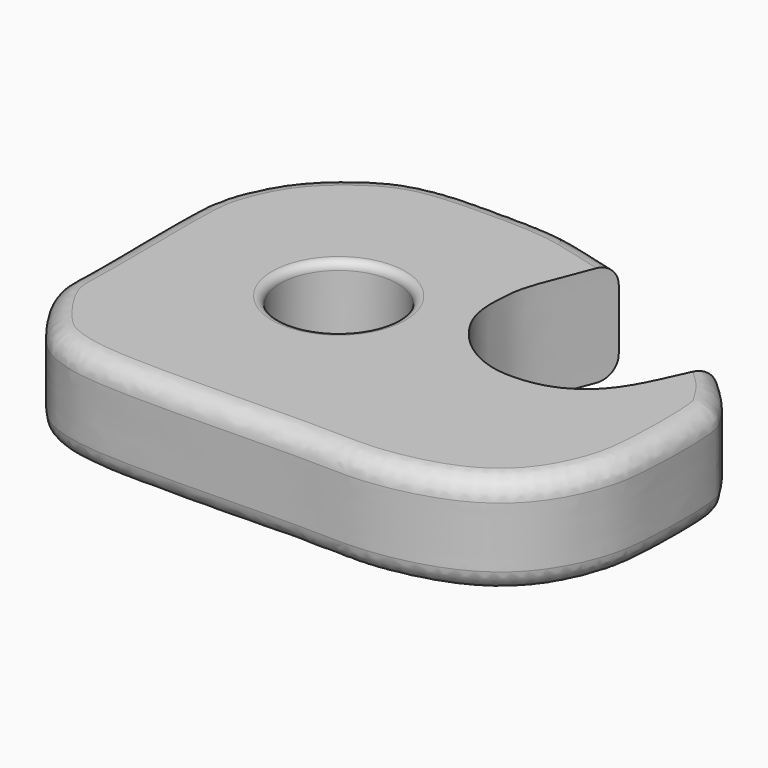
from build123d import *

# Parameters (mm, degrees)
F0_R     = 14.4754712181
F1_DEPTH = 25
F2_R     = 5
F3_R     = 2


with BuildPart() as f1:
    # F0 (on Top) → F1 (new body)
    with BuildSketch(Plane.XY):
        with BuildLine():
            add(Edge.make_bspline(
                [(4.7748561241, 37.0201033496), (1.8727595404, 29.1179646637), (-2.9520116751, 17.9431651207), (-3.3954410177, 12.5793787294), (-3.8071188973, 7.0032014822), (-2.9373384689, 1.6316462754), (-0.6202760255, -2.674310752), (2.3822429436, -6.5357445519), (6.1668697528, -9.7114229849), (10.602603783, -12.05921425), (15.8641316415, -13.4566744805), (22.5388029859, -13.2153438488), (28.2399223964, -11.6976770266), (33.1166668127, -8.7165652858), (36.6710528234, -5.1063898982), (40.3178554583, 0.2360357339), (44.1224099682, 9.0600683626), (46.6542359817, 14.6099540463)],
                knots=[0, 0, 0, 0, 0.1184466174, 0.1765135306, 0.2361345285, 0.2963530059, 0.3530939828, 0.4100083101, 0.4672157798, 0.5246310732, 0.5847048161, 0.651176237, 0.7141127993, 0.775218742, 0.8320476108, 0.8962180189, 1, 1, 1, 1], degree=3))
            add(Edge.make_bspline(
                [(47.3992715806, 14.408958469), (49.5581893602, 12.4293635752), (53.0552771378, 9.14091091), (55.873000337, 4.1728539766), (58.0743199218, 1.4042803534), (57.860107885, -21.4624474724), (56.0155753338, -30.8248650048), (50.6028118678, -43.2032629444), (38.5946445224, -53.9006460259), (17.5542269329, -58.7848208722), (1.8947153131, -57.2572408539), (-48.4788210559, -59.4518328809), (-60.1063658028, -55.7026316627), (-65.7202395809, -52.887305593), (-75.7818557148, -39.1486573699), (-74.5109896884, -29.1899746736), (-75.5520721833, 5.2121806053), (-73.7558927727, 13.4740548272), (-68.2744464695, 26.2721216828), (-56.4052432789, 36.1092530167), (-48.4018948612, 39.8969175531), (-40.2520257831, 41.5180153708), (-29.7568874334, 41.8111730776), (-19.7296486967, 41.7643519531), (-9.3130325779, 41.1205361444), (-0.2326000752, 38.2673542099), (4.7748561241, 37.0201033496)],
                knots=[0, 0, 0, 0, 0.0326111141, 0.0587556715, 0.0801046744, 0.133814265, 0.1716835185, 0.2121781721, 0.2581911555, 0.3094700605, 0.3580706974, 0.4393602896, 0.4787102265, 0.5065811362, 0.5514958373, 0.5903021331, 0.6566719682, 0.6916657518, 0.7331790655, 0.7783952394, 0.8123276102, 0.8450064218, 0.8823187216, 0.9187526227, 0.9556883694, 1, 1, 1, 1], degree=3))
            add(Edge.make_bspline(
                [(46.6542359817, 14.6099540463), (46.7139919849, 14.7342493796), (47.3395155774, 14.2846631356), (47.3992715806, 14.408958469)],
                knots=[0, 0, 0, 0, 0.7716717345, 0.7716717345, 0.7716717345, 0.7716717345], degree=3))
        make_face()
        with Locations((-28.6872740835, -7.8522199765)):
            Circle(F0_R, mode=Mode.SUBTRACT)
    extrude(amount=F1_DEPTH)

    # F2
    f2_edges = [f1.edges().sort_by_distance(p)[0] for p in [
        (-55.074943, -57.039955, 25),
        (-55.074943, -57.039955, 0),
    ]]
    fillet(f2_edges, radius=F2_R)

    # F3
    f3_edges = [f1.edges().sort_by_distance(p)[0] for p in [
        (-14.211803, -7.85222, 12.5),
        (-43.162745, -7.85222, 0),
        (-43.162745, -7.85222, 25),
    ]]
    fillet(f3_edges, radius=F3_R)


solid = f1.part
